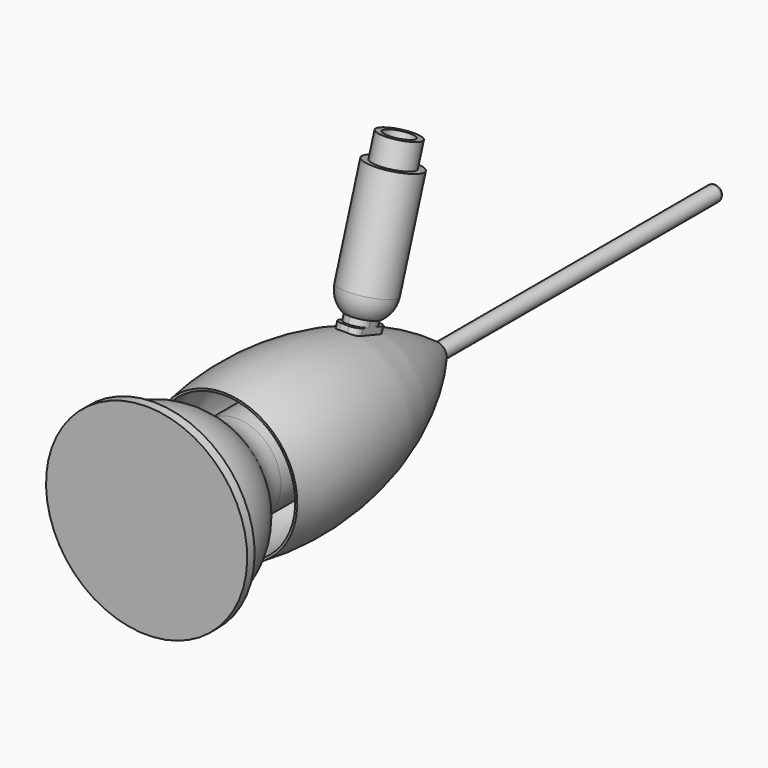
from build123d import *

# Parameters (mm, degrees)
F2_T           = -0.508
F3_R           = 1.905
F4_DEPTH       = 87
F5_R           = 1
F6_R           = 1
F7_DEPTH       = 2.95
F8_R           = 2.94999
F9_R           = 2
F10_R          = 0.3
F16_DEPTH      = 10
F17_R          = 1.99999
F18_R          = 1
F19_DEPTH      = 5.5
F19_DEPTH_BACK = 5.5
F20_R          = 4.9
F20_R_2        = 3.5
F21_DEPTH      = 6
F25_SIZE       = 3


# Not quite as in the source:
# - a fillet or chamfer is up to 0.001 mm smaller than in the source, because OpenCascade refuses the exact size


with BuildPart() as f1:
    # F0 (on Right) → F1 (revolve)
    with BuildSketch(Plane.YZ):
        with BuildLine():
            Line((66, 0), (66, 2.625))
            ThreePointArc((66, 2.625), (34.5943584168, 17.1720699525), (0, 18.25))
            Line((0, 18.25), (0, 0))
            Line((0, 0), (66, 0))
        make_face()
    revolve(axis=Axis((0, 80.7073935866, 0), (0, 1, 0)))

    # F2
    f2_openings = [f1.faces().sort_by_distance(p)[0] for p in [
        (0, 0, 0),
    ]]
    offset(amount=F2_T, openings=f2_openings, kind=Kind.INTERSECTION)

    # F3 (on face) → F4 (join)
    with BuildSketch(Plane(origin=(0, 66, 0), x_dir=(-1, 0, 0), z_dir=(0, 1, 0))):
        Circle(F3_R)
    extrude(amount=F4_DEPTH)

    # F5
    f5_edges = [f1.edges().sort_by_distance(p)[0] for p in [
        (1.905, 153, 0),
    ]]
    fillet(f5_edges, radius=F5_R)

    # F6 (on Right) → F7 (join, symmetric)
    with BuildSketch(Plane.YZ):
        with BuildLine():
            Line((37.6510369808, 17.8326149775), (36.9401659304, 15.6978638563))
            Line((36.9401659304, 15.6978638563), (46.4279486915, 12.5384369655))
            Line((46.4279486915, 12.5384369655), (47.1388197419, 14.6731880867))
            Line((47.1388197419, 14.6731880867), (46.1900414658, 14.9891307758))
            Line((46.1900414658, 14.9891307758), (48.3226546171, 21.3933841395))
            ThreePointArc((48.3226546171, 21.3933841395), (45.791312269, 26.4522680003), (40.7324284082, 23.9209256522))
            Line((40.7324284082, 23.9209256522), (38.5998152569, 17.5166722884))
            Line((38.5998152569, 17.5166722884), (37.6510369808, 17.8326149775))
        make_face()
        with Locations((44.5275415126, 22.6571548959)):
            Circle(F6_R, mode=Mode.SUBTRACT)
    extrude(amount=F7_DEPTH, both=True)

    # F8 (radius 2.95 in the source; OpenCascade refuses exactly that, so slightly less here)
    f8_edges = [f1.edges().sort_by_distance(p)[0] for p in [
        (2.95, 47.256348, 18.191257),
        (-2.95, 47.256348, 18.191257),
        (2.95, 39.666122, 20.718799),
        (-2.95, 39.666122, 20.718799),
        (2.95, 45.791312, 26.452268),
        (-2.95, 45.791312, 26.452268),
    ]]
    fillet(f8_edges, radius=F8_R)

    # F9
    f9_edges = [f1.edges().sort_by_distance(p)[0] for p in [
        (2.95, 46.870144, 13.866354),
        (-2.95, 46.870144, 13.866354),
        (2.95, 37.390196, 17.049307),
        (-2.95, 37.390196, 17.049307),
    ]]
    fillet(f9_edges, radius=F9_R)

    # F10
    f10_edges = [f1.edges().sort_by_distance(p)[0] for p in [
        (0, 66, -2.625),
    ]]
    fillet(f10_edges, radius=F10_R)


with BuildPart() as f13:
    # F12 (on Right) → F13 (revolve)
    with BuildSketch(Plane.YZ):
        with BuildLine():
            Line((52.5840800842, 46.8510009367), (46.4170212895, 48.9046284157))
            Line((46.4170212895, 48.9046284157), (38.3604827179, 24.7107823749))
            ThreePointArc((38.3604827179, 24.7107823749), (38.7146385025, 19.7485197186), (42.4739140336, 16.4900961012))
            Line((42.4739140336, 16.4900961012), (42.7898567227, 17.4388743773))
            ThreePointArc((42.7898567227, 17.4388743773), (39.6089312733, 20.1960020536), (39.309260994, 24.3948396858))
            Line((39.309260994, 24.3948396858), (46.5759428429, 46.2167400363))
            Line((46.5759428429, 46.2167400363), (51.7942233615, 44.4790552464))
            Line((51.7942233615, 44.4790552464), (52.5840800842, 46.8510009367))
        make_face()
    revolve(axis=Axis((0, 44.2094259116, 21.7018513488), (0, 0.3159426891, 0.9487782761)))

    # F15 (on line) → F16 (cut)
    with BuildSketch(Plane(origin=(0, 8.7088867891, 26.1528526538), x_dir=(1, 0, 0), z_dir=(0, 0.3159426891, 0.9487782761))):
        with BuildLine():
            Line((-4, 45.0884016311), (-4, 35.0884016311))
            ThreePointArc((-4, 35.0884016311), (0, 31.0884016311), (4, 35.0884016311))
            Line((4, 35.0884016311), (4, 45.0884016311))
            Line((4, 45.0884016311), (-4, 45.0884016311))
        make_face()
    extrude(amount=F16_DEPTH, mode=Mode.SUBTRACT)

    # F17 (radius 2 in the source; OpenCascade refuses exactly that, so slightly less here)
    f17_edges = [f13.edges().sort_by_distance(p)[0] for p in [
        (-4, 49.380728, 23.14902),
        (4, 49.380728, 23.14902),
    ]]
    fillet(f17_edges, radius=F17_R)

    # F18 (on Right) → F19 (join, two sides)
    with BuildSketch(Plane.YZ) as f19_sk:
        with Locations((44.5275415126, 22.6571548959)):
            Circle(F18_R)
    extrude(amount=F19_DEPTH)
    extrude(f19_sk.sketch, amount=-F19_DEPTH_BACK)

    # F20 (on face) → F21 (join)
    with BuildSketch(Plane(origin=(0, 19.2929668732, 57.9369249035), x_dir=(1, 0, 0), z_dir=(0, 0.3159426891, 0.9487782761))):
        with Locations((0, 35.0884016311)):
            Circle(F20_R)
        with Locations((0, 35.0884016311)):
            Circle(F20_R_2, mode=Mode.SUBTRACT)
    extrude(amount=F21_DEPTH)


with BuildPart() as f24:
    # F23 (on Right) → F24 (revolve)
    with BuildSketch(Plane.YZ):
        with BuildLine():
            Line((-24, 0), (24, 0))
            Line((24, 0), (24, 11))
            Line((24, 11), (4, 11))
            ThreePointArc((4, 11), (-0.6261429599, 12.0112818584), (-4.4083440661, 14.8606404662))
            ThreePointArc((-4.4083440661, 14.8606404662), (-12.186394023, 20.7203113228), (-21.7, 22.8))
            Line((-21.7, 22.8), (-21.7, 25))
            Line((-21.7, 25), (-24, 25))
            Line((-24, 25), (-24, 0))
        make_face()
    revolve(axis=Axis((0, 12, 0), (0, 1, 0)))

    # F25
    f25_edges = [f24.edges().sort_by_distance(p)[0] for p in [
        (0, 24, -11),
    ]]
    chamfer(f25_edges, length=F25_SIZE)


solid = Compound([f1.part, f13.part, f24.part])
